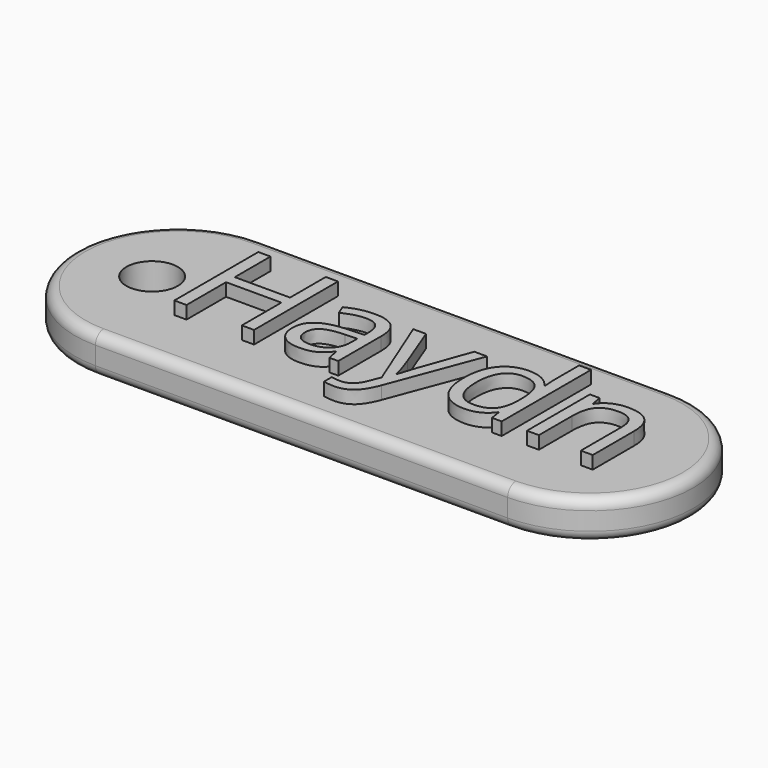
from build123d import *

# Parameters (mm, degrees)
F0_R         = 5
F1_DEPTH     = 7.5
F2_R         = 2
F3_TEXT_SIZE = 28.5326128101
F4_DEPTH     = 2.5


# Not quite as in the source:
# - Text() gives the source's letters only with a copy of the font that has no kerning and outlines rounded to 1/6400 em; it was checked with that copy


with BuildPart() as f1:
    # F0 (on Top) → F1 (new body)
    with BuildSketch(Plane.XY):
        with BuildLine():
            Line((-38.0154633522, -38.1693914306), (41.9845366478, -38.1693914306))
            ThreePointArc((41.9845366478, -38.1693914306), (61.9845366478, -18.1693914306), (41.9845366478, 1.8306085694))
            Line((41.9845366478, 1.8306085694), (-38.0154633522, 1.8306085694))
            ThreePointArc((-38.0154633522, 1.8306085694), (-58.0154633522, -18.1693914306), (-38.0154633522, -38.1693914306))
        make_face()
        with Locations((-43.0154633522, -18.1693914306)):
            Circle(F0_R, mode=Mode.SUBTRACT)
    extrude(amount=F1_DEPTH)

    # F2
    f2_edges = [f1.edges().sort_by_distance(p)[0] for p in [
        (1.984537, 1.830609, 7.5),
        (1.984537, -38.169391, 0),
    ]]
    fillet(f2_edges, radius=F2_R)

    # F3 (on face) → F4 (join)
    with BuildSketch(Plane.XY.offset(7.5)):
        with Locations((-35.2482311428, -25.9882612154)):
            Text('Haydn', F3_TEXT_SIZE, font='Open Sans', text_align=(TextAlign.LEFT, TextAlign.BOTTOM))
    extrude(amount=F4_DEPTH)


solid = f1.part
